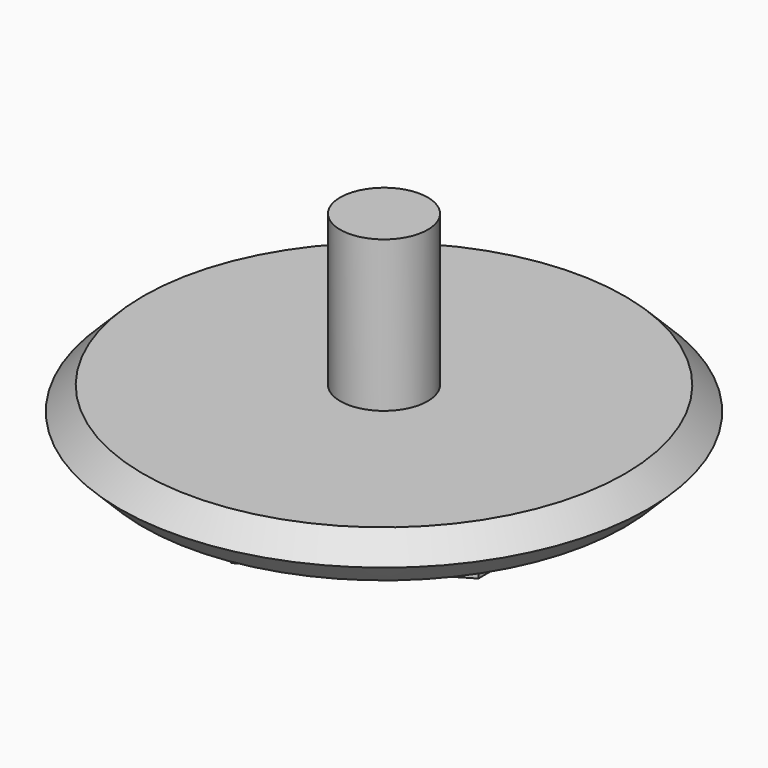
from build123d import *

# Parameters (mm, degrees)
F0_R     = 19.05
F1_DEPTH = 3.302
F2_R     = 3.0940455734
F3_DEPTH = 10.668
F4_SIZE  = 2.032
F7_DEPTH = 2.286


# Not quite as in the source:
# - a fillet or chamfer that OpenCascade refuses, or shapes differently, is made with other operations: its cross-section is extruded or revolved along the edge and cut away or added


with BuildPart() as f1:
    # F0 (on Top) → F1 (new body)
    with BuildSketch(Plane.XY):
        Circle(F0_R)
    extrude(amount=F1_DEPTH)

    # F2 (on face) → F3 (join)
    with BuildSketch(Plane.XY.offset(3.302)):
        Circle(F2_R)
    extrude(amount=F3_DEPTH)

    # F4
    f4_edges = [f1.edges().sort_by_distance(p)[0] for p in [
        (-19.05, 0, 3.302),
    ]]
    chamfer(f4_edges, length=F4_SIZE)

    # F5: chamfer of 2.032 on 1 edges, made by hand

    # F5_s1 → F5_t2 (revolve, cut)
    with BuildSketch(Plane.XZ):
        Polygon((19.05, 2.032), (17.018, 0), (19.05, 0), align=None)
    revolve(axis=Axis((0, 0, 0), (0, 0, 1)), mode=Mode.SUBTRACT)

    # F6 (on face) → F7 (join)
    with BuildSketch(Plane(origin=(0, 0, 0), x_dir=(1, 0, 0), z_dir=(0, 0, -1))):
        Polygon((-10.1241571829, 7.50669837), (-11.5505903959, 6.6151777282), (-11.4901715756, -3.6598756731), (-2.9577685054, -8.7351842692), (4.4179176912, -4.5286850072), (4.4179176912, -6.1632911675), (-2.9577685054, -10.3697904294), (-11.5558920335, -5.255389493), (-11.5558920335, -6.9493146705), (-2.9577685054, -12.0637156069), (5.9589991364, -7.1465903893), (5.9589991364, 1.4732169604), (7.414681837, 0.6073367549), (7.414681837, -7.955128327), (-1.1376237962, -13.150122948), (0.1876302122, -13.7365777045), (8.8004540583, -8.6443684995), (8.8004540583, 1.404343208), (1.6391712, 5.6640716984), (3.2676828559, 6.4783277921), (10.5352541432, 2.4422151037), (10.5352541432, -7.7702743001), (11.6456285548, -6.8170730956), (11.6456285548, 3.0340532394), (3.4269623458, 7.9227425003), (-4.1806832887, 4.1189184412), (-4.1806832887, 5.604787264), (3.0703544617, 9.7057837993), (11.8158220797, 5.0698746927), (11.8158220797, 6.4297318659), (3.0109197833, 11.667130515), (-5.9344387757, 6.6151777282), (-5.9344387757, -2.0622941665), (-7.0335506462, -1.408512122), (-7.0335506462, 7.50669837), (1.4481722892, 12.6481941369), (0, 13.5096069425), (-8.5194194689, 8.338784799), (-8.5194194689, -2.0622941665), (-1.6249895561, -6.1632911675), (-3.0514232349, -6.8765082397), (-10.1241571829, -2.7755110059), align=None)
        Polygon((0, -5.4471737376), (-4.3624499813, -2.7635633014), (-4.3624499813, 2.5107886177), (0, 4.998779855), (4.4179176912, 2.3708806043), (4.4179176912, -2.7635630686), align=None, mode=Mode.SUBTRACT)
    extrude(amount=F7_DEPTH)


solid = f1.part
